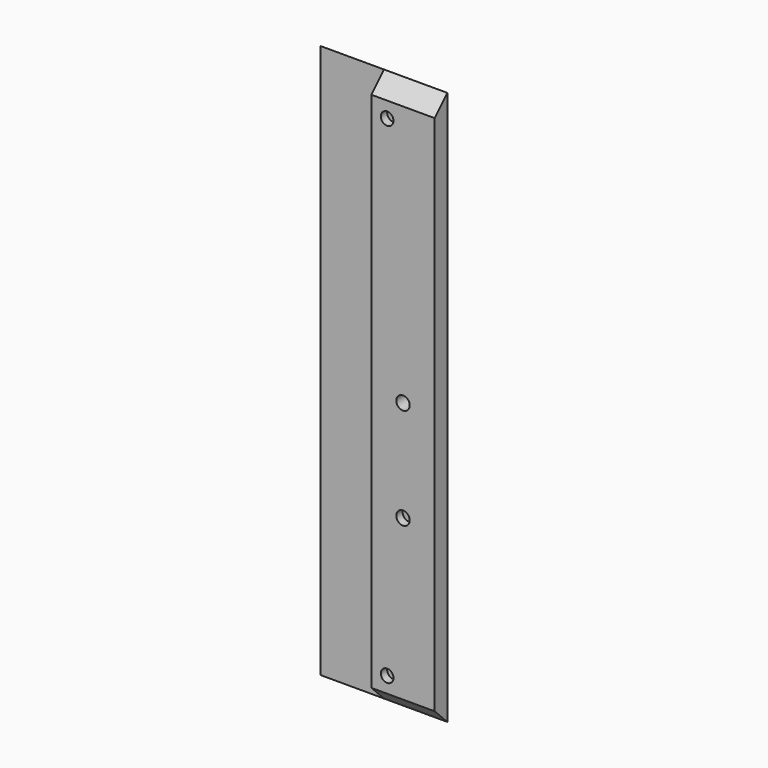
from build123d import *

# Parameters (mm, degrees)
F0_W      = 40
F0_H      = 10
F1_DEPTH  = 350
F2_SIZE   = 9.99999
F3_SIZE   = 9.99999
F4_W      = 40
F4_H      = 10
F5_DEPTH  = 350
F6_SIZE   = 9.99999
F7_SIZE   = 9.99999
F8_R      = 4.25
F9_DEPTH  = 10.001
F10_R     = 2
F10_R_2   = 4
F11_DEPTH = 5
F12_R     = 4.25
F12_R_2   = 4
F13_DEPTH = 5


# Not quite as in the source:
# - a fillet or chamfer is up to 0.001 mm smaller than in the source, because OpenCascade refuses the exact size


with BuildPart() as f1:
    # F0 (on Top) → F1 (new body)
    with BuildSketch(Plane.XY):
        with Locations((-20, 5)):
            Rectangle(F0_W, F0_H)
    extrude(amount=F1_DEPTH)

    # F2 (size 10 in the source; OpenCascade refuses exactly that, so slightly less here)
    f2_edges = [f1.edges().sort_by_distance(p)[0] for p in [
        (-20, 10, 350),
    ]]
    chamfer(f2_edges, length=F2_SIZE)

    # F3 (size 10 in the source; OpenCascade refuses exactly that, so slightly less here)
    f3_edges = [f1.edges().sort_by_distance(p)[0] for p in [
        (-20, 10, 0),
    ]]
    chamfer(f3_edges, length=F3_SIZE)

    # F10 (on face) → F11 (cut)
    with BuildSketch(Plane(origin=(0, 10, 0), x_dir=(-1, 0, 0), z_dir=(0, 1, 0))):
        with Locations((20, 305)):
            Circle(F10_R)
        with Locations((10, 330)):
            Circle(F10_R_2)
        with Locations((10, 20)):
            Circle(F10_R_2)
    extrude(amount=-F11_DEPTH, mode=Mode.SUBTRACT)


with BuildPart() as f5:
    # F4 (on Top) → F5 (new body)
    with BuildSketch(Plane.XY):
        with Locations((20, -5)):
            Rectangle(F4_W, F4_H)
    extrude(amount=F5_DEPTH)

    # F6 (size 10 in the source; OpenCascade refuses exactly that, so slightly less here)
    f6_edges = [f5.edges().sort_by_distance(p)[0] for p in [
        (20, -10, 0),
    ]]
    chamfer(f6_edges, length=F6_SIZE)

    # F7 (size 10 in the source; OpenCascade refuses exactly that, so slightly less here)
    f7_edges = [f5.edges().sort_by_distance(p)[0] for p in [
        (20, -10, 350),
    ]]
    chamfer(f7_edges, length=F7_SIZE)

    # F8 (on face) → F9 (cut, through all)
    with BuildSketch(Plane(origin=(0, 0, 0), x_dir=(-1, 0, 0), z_dir=(0, 1, 0))):
        with Locations((-20, 175)):
            Circle(F8_R)
    extrude(amount=-F9_DEPTH, mode=Mode.SUBTRACT)

    # F12 (on face) → F13 (cut)
    with BuildSketch(Plane.XZ.offset(10)):
        with Locations((20, 111)):
            Circle(F12_R)
        with Locations((10, 20)):
            Circle(F12_R_2)
        with Locations((10, 330)):
            Circle(F12_R_2)
    extrude(amount=-F13_DEPTH, mode=Mode.SUBTRACT)


solid = Compound([f1.part, f5.part])
